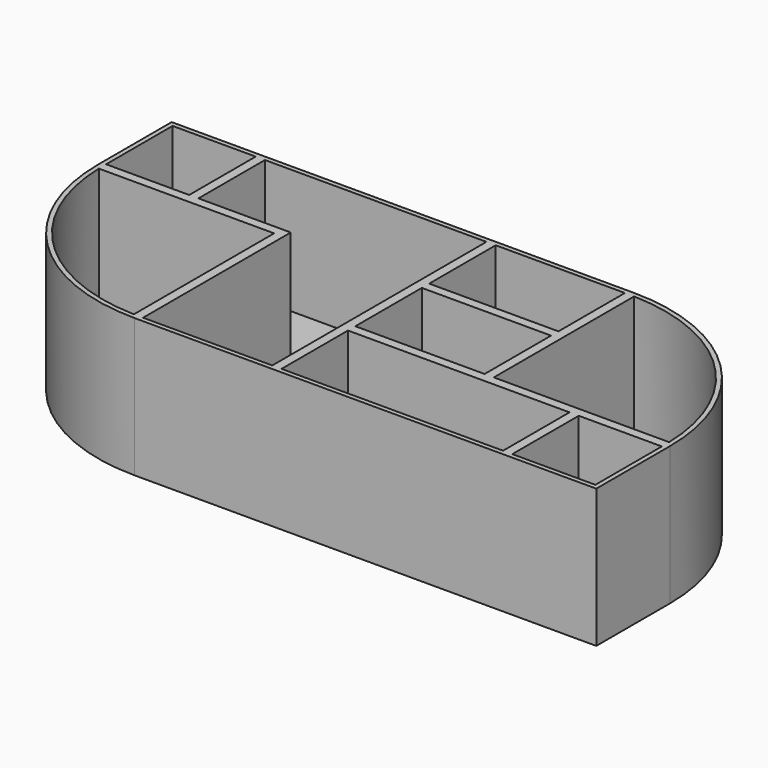
from build123d import *

# Parameters (mm, degrees)
F0_W     = 20
F0_H     = 20
F0_W_2   = 18
F0_H_2   = 18
F0_W_3   = 30
F0_W_4   = 28
F1_DEPTH = 30
F2_DEPTH = 3


# Not quite as in the source:
# - a feature names something its author has since deleted; it is built from what else it names


with BuildPart() as f1:
    # F0 (on Top) → F1 (new body)
    with BuildSketch(Plane.XY):
        with Locations((60, -20)):
            Rectangle(F0_W, F0_H)
        with Locations((60, -20)):
            Rectangle(F0_W_2, F0_H_2, mode=Mode.SUBTRACT)
        Polygon((0, -30), (50, -30), (50, -10), (30, -10), (0, -10), align=None)
        Polygon((49, -11), (49, -29), (1, -29), (1, -11), (30, -11), align=None, mode=Mode.SUBTRACT)
        with BuildLine():
            Line((50, -10), (70, -10))
            ThreePointArc((70, -10), (58.2842712475, 18.2842712475), (30, 30))
            Line((30, 30), (30, 10))
            Line((30, 10), (30, -10))
            Line((30, -10), (50, -10))
        make_face()
        with BuildLine():
            Line((68.9871769817, -8.9999996126), (31.0000003874, -8.9999996126))
            Line((31.0000003874, -8.9999996126), (31.0000003874, 10))
            Line((31.0000003874, 10), (31.0000003874, 28.9871769817))
            ThreePointArc((31.0000003874, 28.9871769817), (57.5771641923, 17.5771641923), (68.9871769817, -8.9999996126))
        make_face(mode=Mode.SUBTRACT)
        Polygon((-30, -30), (0, -30), (0, -10), (0, 10), (0, 30), (-50, 30), (-50, 10), (-30, 10), (-30, -29.9919991921), (-30, -29.9959995961), align=None)
        Polygon((-49, 29), (-1, 29), (-1, -29), (-29, -29), (-29, 11), (-49, 11), align=None, mode=Mode.SUBTRACT)
        with Locations((15, 20)):
            Rectangle(F0_W_3, F0_H)
        with Locations((15, 20)):
            Rectangle(F0_W_4, F0_H_2, mode=Mode.SUBTRACT)
        with Locations((15, 0)):
            Rectangle(F0_W_3, F0_H)
        with Locations((15, 0)):
            Rectangle(F0_W_4, F0_H_2, mode=Mode.SUBTRACT)
        Polygon((-50, 10), (-50, 30), (-70, 30), (-70, 10), (-69.9919991921, 10), align=None)
        with Locations((-60, 20)):
            Rectangle(F0_W_2, F0_H_2, mode=Mode.SUBTRACT)
        with BuildLine():
            ThreePointArc((-69.9919991921, 10), (-58.278613822, -18.278613822), (-30, -29.9919991921))
            Line((-30, -29.9919991921), (-30, 10))
            Line((-30, 10), (-50, 10))
            Line((-50, 10), (-69.9919991921, 10))
        make_face()
        with BuildLine():
            ThreePointArc((-30.999999342, -28.9791746145), (-57.5715075061, -17.5715075061), (-68.9791746145, 9.000000658))
            Line((-68.9791746145, 9.000000658), (-50, 9.000000658))
            Line((-50, 9.000000658), (-30.999999342, 9.000000658))
            Line((-30.999999342, 9.000000658), (-30.999999342, -28.9791746145))
        make_face(mode=Mode.SUBTRACT)
    extrude(amount=F1_DEPTH)

    # F0 (on Top) → F2 (join)
    with BuildSketch(Plane.XY):
        with Locations((-60, 20)):
            Rectangle(F0_W_2, F0_H_2)
        Polygon((-1, -29), (-1, 29), (-49, 29), (-49, 11), (-29, 11), (-29, -29), align=None)
        with BuildLine():
            Line((-50, 9.000000658), (-68.9791746145, 9.000000658))
            ThreePointArc((-68.9791746145, 9.000000658), (-57.5715075061, -17.5715075061), (-30.999999342, -28.9791746145))
            Line((-30.999999342, -28.9791746145), (-30.999999342, 9.000000658))
            Line((-30.999999342, 9.000000658), (-50, 9.000000658))
        make_face()
        with Locations((15, 0)):
            Rectangle(F0_W_4, F0_H_2)
        with Locations((15, 20)):
            Rectangle(F0_W_4, F0_H_2)
        with BuildLine():
            Line((31.0000003874, 10), (31.0000003874, -8.9999996126))
            Line((31.0000003874, -8.9999996126), (68.9871769817, -8.9999996126))
            ThreePointArc((68.9871769817, -8.9999996126), (57.5771641923, 17.5771641923), (31.0000003874, 28.9871769817))
            Line((31.0000003874, 28.9871769817), (31.0000003874, 10))
        make_face()
        Polygon((1, -29), (49, -29), (49, -11), (30, -11), (1, -11), align=None)
        with Locations((60, -20)):
            Rectangle(F0_W_2, F0_H_2)
    extrude(amount=F2_DEPTH)


solid = f1.part
